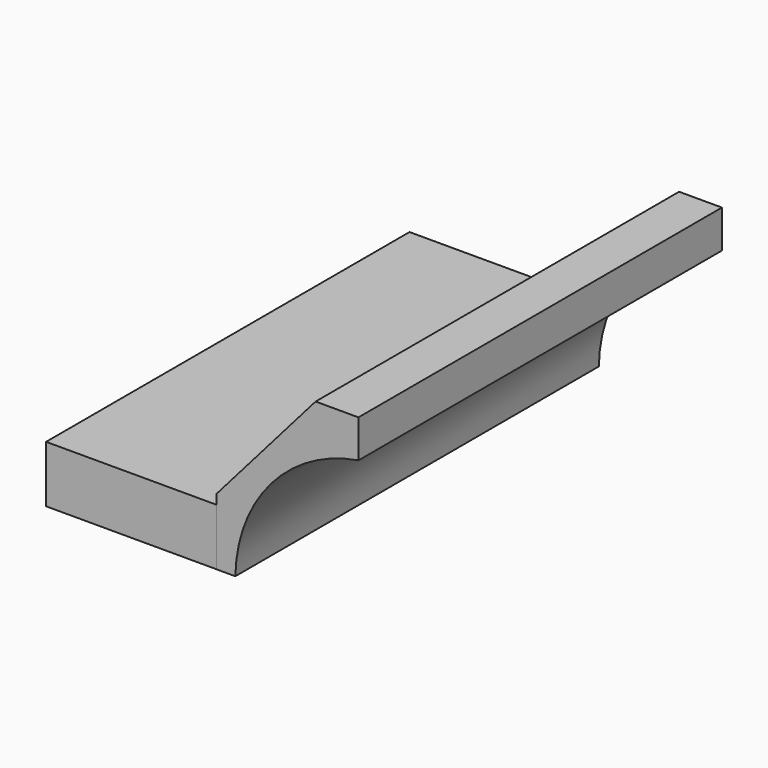
from build123d import *

# Parameters (mm, degrees)
F0_W     = 57.15
F0_H     = 19.05
F1_DEPTH = 152.4000018835
F2_DEPTH = 152.4253934622


# Not quite as in the source:
# - ends of sketch curves that miss each other by under 0.0002 mm in the source are joined


with BuildPart() as f1:
    # F0 (on Front) → F1 (new body)
    with BuildSketch(Plane.XZ):
        with Locations((-23.829137, -20.6585566)):
            Rectangle(F0_W, F0_H)
    extrude(amount=F1_DEPTH)

    # F0 (on Front) → F2 (join)
    with BuildSketch(Plane.XZ):
        with BuildLine():
            Line((4.745863, -11.1335566), (4.745863, -30.1835566))
            Line((4.745863, -30.1835566), (11.100308, -30.1835566))
            ThreePointArc((11.100308, -30.1835566), (23.1263213226, 1.121334901), (52.4041128155, 17.4746845664))
            Line((52.4041128155, 17.4746845664), (52.4041116, 30.1835566))
            Line((52.4041116, 30.1835566), (38.0344934, 30.1835566))
            Line((38.0344934, 30.1835566), (4.745863, -7.9430372))
            Line((4.745863, -7.9430372), (4.745863, -11.1335566))
        make_face()
    extrude(amount=F2_DEPTH)


solid = f1.part
